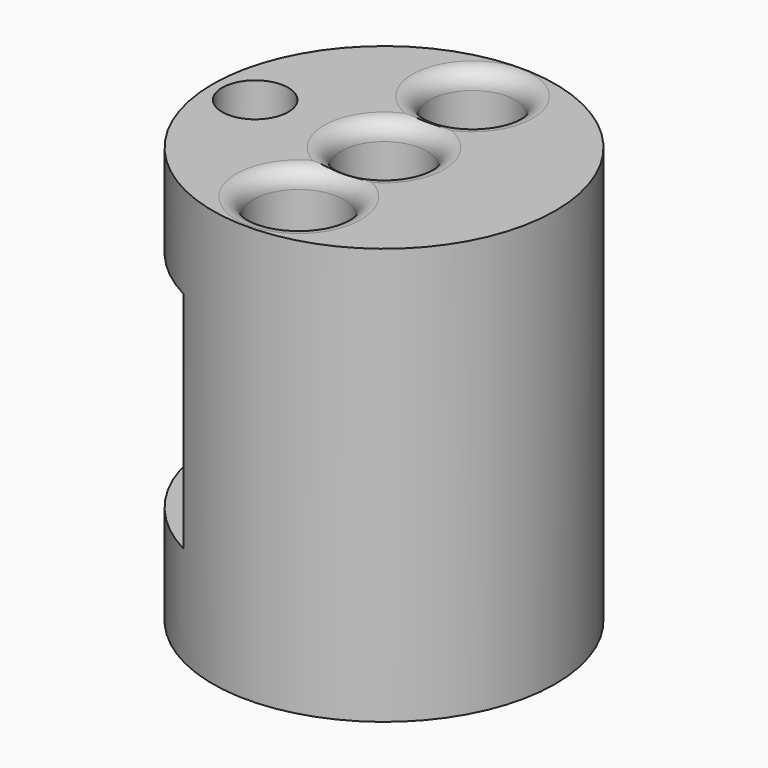
from build123d import *

# Parameters (mm, degrees)
F0_R     = 50.8
F0_R_2   = 13.4110362239
F0_R_3   = 12.7
F1_DEPTH = 61.722
F3_W     = 62.9586838186
F3_H     = 66.4563924074
F4_DEPTH = 93.98
F5_R     = 9.7904939915
F6_DEPTH = 90.17


# Not quite as in the source:
# - a fillet or chamfer that OpenCascade refuses, or shapes differently, is made with other operations: its cross-section is extruded or revolved along the edge and cut away or added


with BuildPart() as f1:
    # F0 (on Top) → F1 (new body, symmetric)
    with BuildSketch(Plane.XY):
        Circle(F0_R)
        with Locations((0, -31.6250808537)):
            Circle(F0_R_2, mode=Mode.SUBTRACT)
        Circle(F0_R_3, mode=Mode.SUBTRACT)
        with Locations((0, 32.7909812331)):
            Circle(F0_R_3, mode=Mode.SUBTRACT)
    extrude(amount=F1_DEPTH, both=True)

    # F2: fillet of radius 5.08 on 9 edges, made by hand

    # F2_s1 → F2_t2 (revolve, cut)
    with BuildSketch(Plane.XZ.offset(31.6250808537)):
        with BuildLine():
            ThreePointArc((18.4910362239, 61.722), (14.8989337755, 60.2341024484), (13.4110362239, 56.642))
            Line((13.4110362239, 56.642), (13.4110362239, 61.722))
            Line((13.4110362239, 61.722), (18.4910362239, 61.722))
        make_face()
    revolve(axis=Axis((0, -31.6250808537, 61.722), (0, 0, 1)), mode=Mode.SUBTRACT)

    # F2_s3 → F2_t4 (revolve, cut)
    with BuildSketch(Plane.XZ.offset(31.6250808537)):
        with BuildLine():
            ThreePointArc((13.4110362239, -56.642), (14.8989337755, -60.2341024484), (18.4910362239, -61.722))
            Line((18.4910362239, -61.722), (13.4110362239, -61.722))
            Line((13.4110362239, -61.722), (13.4110362239, -56.642))
        make_face()
    revolve(axis=Axis((0, -31.6250808537, -61.722), (0, 0, 1)), mode=Mode.SUBTRACT)

    # F2_s5 → F2_t6 (revolve, cut)
    with BuildSketch(Plane.XZ):
        with BuildLine():
            ThreePointArc((17.78, 61.722), (14.1878975516, 60.2341024484), (12.7, 56.642))
            Line((12.7, 56.642), (12.7, 61.722))
            Line((12.7, 61.722), (17.78, 61.722))
        make_face()
    revolve(axis=Axis((0, 0, 61.722), (0, 0, 1)), mode=Mode.SUBTRACT)

    # F2_s7 → F2_t8 (revolve, cut)
    with BuildSketch(Plane.XZ):
        with BuildLine():
            ThreePointArc((12.7, -56.642), (14.1878975516, -60.2341024484), (17.78, -61.722))
            Line((17.78, -61.722), (12.7, -61.722))
            Line((12.7, -61.722), (12.7, -56.642))
        make_face()
    revolve(axis=Axis((0, 0, -61.722), (0, 0, 1)), mode=Mode.SUBTRACT)

    # F2_s9 → F2_t10 (revolve, cut)
    with BuildSketch(Plane.XZ.offset(-32.7909812331)):
        with BuildLine():
            ThreePointArc((17.78, 61.722), (14.1878975516, 60.2341024484), (12.7, 56.642))
            Line((12.7, 56.642), (12.7, 61.722))
            Line((12.7, 61.722), (17.78, 61.722))
        make_face()
    revolve(axis=Axis((0, 32.7909812331, 61.722), (0, 0, 1)), mode=Mode.SUBTRACT)

    # F2_s11 → F2_t12 (revolve, cut)
    with BuildSketch(Plane.XZ.offset(-32.7909812331)):
        with BuildLine():
            ThreePointArc((12.7, -56.642), (14.1878975516, -60.2341024484), (17.78, -61.722))
            Line((17.78, -61.722), (12.7, -61.722))
            Line((12.7, -61.722), (12.7, -56.642))
        make_face()
    revolve(axis=Axis((0, 32.7909812331, -61.722), (0, 0, 1)), mode=Mode.SUBTRACT)

    # F3 (on Front) → F4 (cut, symmetric)
    with BuildSketch(Plane.XZ):
        with Locations((-54.7973755747, 1.0201632977)):
            Rectangle(F3_W, F3_H)
    extrude(amount=F4_DEPTH, both=True, mode=Mode.SUBTRACT)

    # F5 (on Top) → F6 (cut)
    with BuildSketch(Plane.XY):
        with Locations((-38.1832793355, 0)):
            Circle(F5_R)
    extrude(amount=F6_DEPTH, mode=Mode.SUBTRACT)


solid = f1.part
